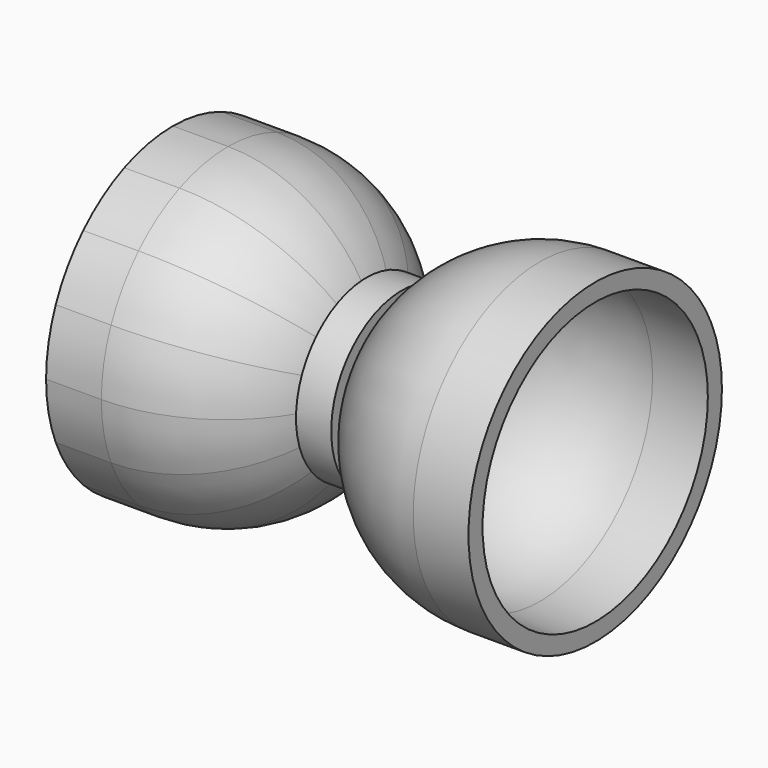
from build123d import *

# Parameters (mm, degrees)
F0_R      = 22.86
F1_DEPTH  = 30.48
F2_T      = -2.54
F3_R      = 19.959955
F4_R      = 22.499955
F7_DEPTH  = 30.48
F8_T      = -2.54
F9_R      = 19.959955
F10_R     = 22.499955
F11_R     = 12.7
F12_DEPTH = 2.54


with BuildPart() as f1:
    # F0 (on Right) → F1 (new body)
    with BuildSketch(Plane.YZ):
        Circle(F0_R)
    extrude(amount=F1_DEPTH)

    # F2
    f2_openings = [f1.faces().sort_by_distance(p)[0] for p in [
        (30.48, 0, 0),
    ]]
    offset(amount=F2_T, openings=f2_openings)

    # F3
    f3_edges = [f1.edges().sort_by_distance(p)[0] for p in [
        (2.54, -20.32, 0),
    ]]
    fillet(f3_edges, radius=F3_R)

    # F4
    f4_edges = [f1.edges().sort_by_distance(p)[0] for p in [
        (0, -22.86, 0),
    ]]
    fillet(f4_edges, radius=F4_R)


with BuildPart() as f7:
    # F6 (on offset) → F7 (new body)
    with BuildSketch(Plane.YZ.offset(-30.48)):
        with BuildLine():
            Line((0, 0), (22.86, 0))
            ThreePointArc((22.86, 0), (22.42075151, 4.4597647613), (21.1198861132, 8.7481432639))
            Line((21.1198861132, 8.7481432639), (0, 0))
        make_face()
        with BuildLine():
            Line((0, 0), (21.1198861132, 8.7481432639))
            ThreePointArc((21.1198861132, 8.7481432639), (19.0073953372, 12.7003355268), (16.1644610179, 16.1644610179))
            Line((16.1644610179, 16.1644610179), (0, 0))
        make_face()
        with BuildLine():
            Line((8.7481432639, 21.1198861132), (0, 0))
            Line((0, 0), (16.1644610179, 16.1644610179))
            ThreePointArc((16.1644610179, 16.1644610179), (12.7003355268, 19.0073953372), (8.7481432639, 21.1198861132))
        make_face()
        with BuildLine():
            Line((0, 22.86), (0, 0))
            Line((0, 0), (8.7481432639, 21.1198861132))
            ThreePointArc((8.7481432639, 21.1198861132), (4.4597647613, 22.42075151), (0, 22.86))
        make_face()
        with BuildLine():
            Line((-8.7481432639, 21.1198861132), (0, 0))
            Line((0, 0), (0, 22.86))
            ThreePointArc((0, 22.86), (-4.4597647613, 22.42075151), (-8.7481432639, 21.1198861132))
        make_face()
        with BuildLine():
            Line((-16.1644610179, 16.1644610179), (0, 0))
            Line((0, 0), (-8.7481432639, 21.1198861132))
            ThreePointArc((-8.7481432639, 21.1198861132), (-12.7003355268, 19.0073953372), (-16.1644610179, 16.1644610179))
        make_face()
        with BuildLine():
            Line((-21.1198861132, 8.7481432639), (0, 0))
            Line((0, 0), (-16.1644610179, 16.1644610179))
            ThreePointArc((-16.1644610179, 16.1644610179), (-19.0073953372, 12.7003355268), (-21.1198861132, 8.7481432639))
        make_face()
        with BuildLine():
            Line((-22.86, 0), (0, 0))
            Line((0, 0), (-21.1198861132, 8.7481432639))
            ThreePointArc((-21.1198861132, 8.7481432639), (-22.42075151, 4.4597647613), (-22.86, 0))
        make_face()
        with BuildLine():
            Line((-21.1198861132, -8.7481432639), (0, 0))
            Line((0, 0), (-22.86, 0))
            ThreePointArc((-22.86, 0), (-22.42075151, -4.4597647613), (-21.1198861132, -8.7481432639))
        make_face()
        with BuildLine():
            Line((-16.1644610179, -16.1644610179), (0, 0))
            Line((0, 0), (-21.1198861132, -8.7481432639))
            ThreePointArc((-21.1198861132, -8.7481432639), (-19.0073953372, -12.7003355268), (-16.1644610179, -16.1644610179))
        make_face()
        with BuildLine():
            Line((-8.7481432639, -21.1198861132), (0, 0))
            Line((0, 0), (-16.1644610179, -16.1644610179))
            ThreePointArc((-16.1644610179, -16.1644610179), (-12.7003355268, -19.0073953372), (-8.7481432639, -21.1198861132))
        make_face()
        with BuildLine():
            Line((0, -22.86), (0, 0))
            Line((0, 0), (-8.7481432639, -21.1198861132))
            ThreePointArc((-8.7481432639, -21.1198861132), (-4.4597647613, -22.42075151), (0, -22.86))
        make_face()
        with BuildLine():
            Line((8.7481432639, -21.1198861132), (0, 0))
            Line((0, 0), (0, -22.86))
            ThreePointArc((0, -22.86), (4.4597647613, -22.42075151), (8.7481432639, -21.1198861132))
        make_face()
        with BuildLine():
            Line((16.1644610179, -16.1644610179), (0, 0))
            Line((0, 0), (8.7481432639, -21.1198861132))
            ThreePointArc((8.7481432639, -21.1198861132), (12.7003355268, -19.0073953372), (16.1644610179, -16.1644610179))
        make_face()
        with BuildLine():
            ThreePointArc((16.1644610179, -16.1644610179), (19.0073953372, -12.7003355268), (21.1198861132, -8.7481432639))
            Line((21.1198861132, -8.7481432639), (0, 0))
            Line((0, 0), (16.1644610179, -16.1644610179))
        make_face()
        with BuildLine():
            ThreePointArc((21.1198861132, -8.7481432639), (22.42075151, -4.4597647613), (22.86, 0))
            Line((22.86, 0), (0, 0))
            Line((0, 0), (21.1198861132, -8.7481432639))
        make_face()
    extrude(amount=F7_DEPTH)

    # F8
    f8_openings = [f7.faces().sort_by_distance(p)[0] for p in [
        (-30.48, 0, 0),
    ]]
    offset(amount=F8_T, openings=f8_openings)

    # F9
    f9_edges = [f7.edges().sort_by_distance(p)[0] for p in [
        (-2.54, -18.773232, 7.776127),
    ]]
    fillet(f9_edges, radius=F9_R)

    # F10
    f10_edges = [f7.edges().sort_by_distance(p)[0] for p in [
        (0, -21.119886, 8.748143),
    ]]
    fillet(f10_edges, radius=F10_R)


with BuildPart() as f12:
    # F11 (on Right) → F12 (new body, symmetric)
    with BuildSketch(Plane.YZ):
        Circle(F11_R)
    extrude(amount=F12_DEPTH, both=True)


solid = Compound([f1.part, f7.part, f12.part])
